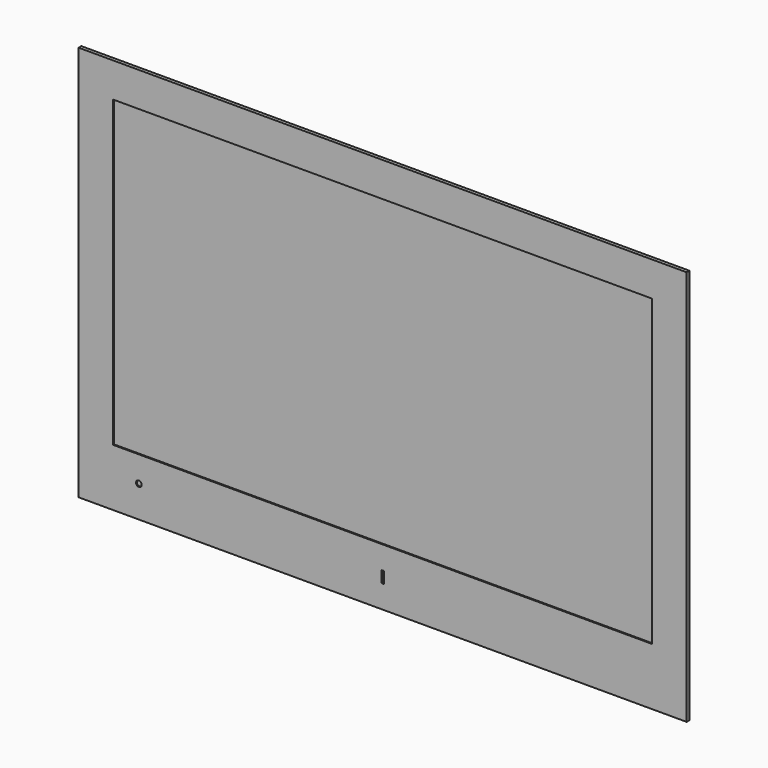
from build123d import *

# Parameters (mm, degrees)
F0_W     = 530
F0_H     = 345
F0_R     = 2.5
F0_W_2   = 2
F0_H_2   = 10
F0_W_3   = 470
F0_H_3   = 265
F1_DEPTH = 3
F2_W     = 470
F2_H     = 265
F2_R     = 2.5
F2_W_2   = 2
F2_H_2   = 10
F3_DEPTH = 1
F4_W     = 390
F4_H     = 295
F4_H_2   = 245
F5_DEPTH = 30


with BuildPart() as f1:
    # F0 (on Front) → F1 (new body)
    with BuildSketch(Plane.XZ):
        Rectangle(F0_W, F0_H)
        with Locations((-212.5, -145)):
            Circle(F0_R, mode=Mode.SUBTRACT)
        with Locations((0, -147.5)):
            Rectangle(F0_W_2, F0_H_2, mode=Mode.SUBTRACT)
        with Locations((0, 10)):
            Rectangle(F0_W_3, F0_H_3, mode=Mode.SUBTRACT)
        with Locations((0, 10)):
            Rectangle(F0_W_3, F0_H_3)
        with Locations((0, -147.5)):
            Rectangle(F0_W_2, F0_H_2)
        with Locations((-212.5, -145)):
            Circle(F0_R)
    extrude(amount=F1_DEPTH)

    # F2 (on face) → F3 (cut)
    with BuildSketch(Plane.XZ.offset(3)):
        with Locations((0, 10)):
            Rectangle(F2_W, F2_H)
        with Locations((-212.5, -145)):
            Circle(F2_R)
        with Locations((0, -147.5)):
            Rectangle(F2_W_2, F2_H_2)
    extrude(amount=-F3_DEPTH, mode=Mode.SUBTRACT)

    # F4 (on face) → F5 (join)
    with BuildSketch(Plane.XZ):
        with Locations((0, -25)):
            Rectangle(F4_W, F4_H)
        Rectangle(F4_W, F4_H_2)
    extrude(amount=-F5_DEPTH)


solid = f1.part
